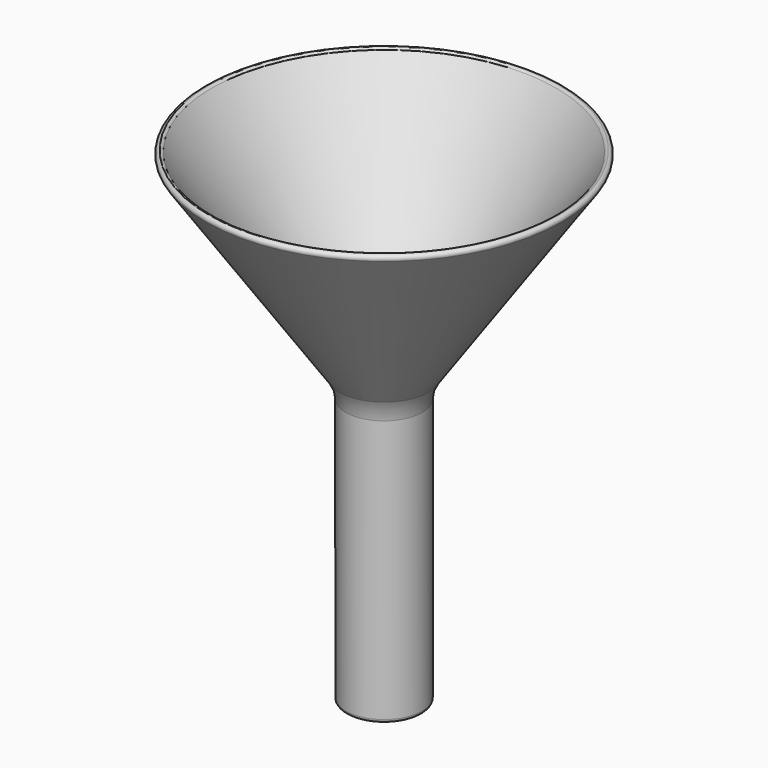
from build123d import *

# Parameters (mm, degrees)
F2_R = 0.99999
F3_R = 5
F4_R = 10


# Not quite as in the source:
# - a fillet or chamfer is up to 0.001 mm smaller than in the source, because OpenCascade refuses the exact size


with BuildPart() as f1:
    # F0 (on Front) → F1 (revolve)
    with BuildSketch(Plane.XZ):
        Polygon((-11, 80), (-11, 0), (-9, 0), (-9, 80.6242772277), (-50.0682082509, 140), (-52.5, 140), align=None)
    revolve(axis=Axis((0, 0, 40), (0, 0, 1)))

    # F2 (radius 1 in the source; OpenCascade refuses exactly that, so slightly less here)
    f2_edges = [f1.edges().sort_by_distance(p)[0] for p in [
        (52.5, 0, 140),
        (50.068208, 0, 140),
        (11, 0, 0),
        (9, 0, 0),
    ]]
    fillet(f2_edges, radius=F2_R)

    # F3
    f3_edges = [f1.edges().sort_by_distance(p)[0] for p in [
        (9, 0, 80.624277),
    ]]
    fillet(f3_edges, radius=F3_R)

    # F4
    f4_edges = [f1.edges().sort_by_distance(p)[0] for p in [
        (11, 0, 80),
    ]]
    fillet(f4_edges, radius=F4_R)


solid = f1.part
